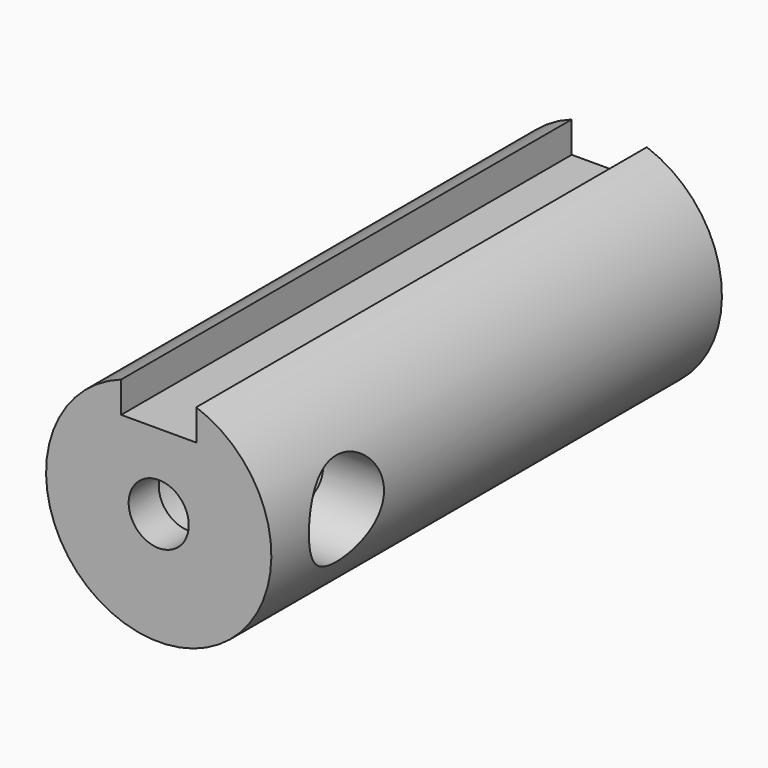
from build123d import *

# Parameters (mm, degrees)
F0_R      = 6
F1_DEPTH  = 30
F2_R      = 2.75
F3_DEPTH  = 30.001
F8_R      = 5
F8_R_2    = 1.6
F9_DEPTH  = 2
F12_W     = 4
F12_H     = 30
F13_DEPTH = 3
F14_R     = 2.5
F15_DEPTH = 3.5


with BuildPart() as f1:
    # F0 (on Front) → F1 (new body)
    with BuildSketch(Plane.XZ):
        Circle(F0_R)
    extrude(amount=F1_DEPTH)

    # F2 (on face) → F3 (cut, through all)
    with BuildSketch(Plane.XZ.offset(30)):
        Circle(F2_R)
    extrude(amount=-F3_DEPTH, mode=Mode.SUBTRACT)

    # F8 (on face) → F9 (join)
    with BuildSketch(Plane.XZ.offset(30)):
        Circle(F8_R)
        Circle(F8_R_2, mode=Mode.SUBTRACT)
    extrude(amount=-F9_DEPTH)

    # F12 (on offset) → F13 (cut)
    with BuildSketch(Plane.XY.offset(4)):
        with Locations((0, -15)):
            Rectangle(F12_W, F12_H)
    extrude(amount=F13_DEPTH, mode=Mode.SUBTRACT)

    # F14 (on offset) → F15 (cut)
    with BuildSketch(Plane.YZ.offset(6)):
        with Locations((-25, 0)):
            Circle(F14_R)
    extrude(amount=-F15_DEPTH, mode=Mode.SUBTRACT)


solid = f1.part
